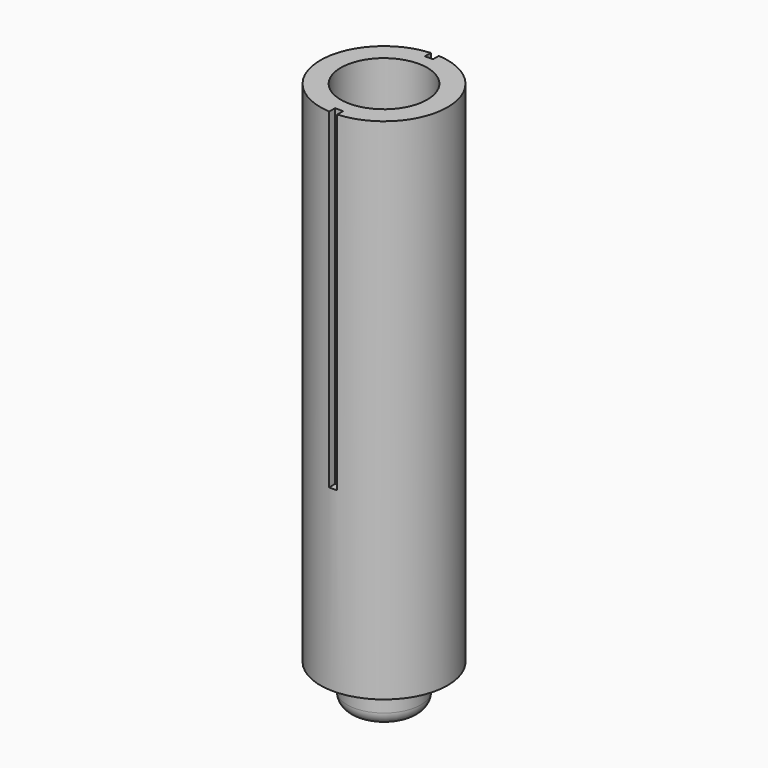
from build123d import *

# Parameters (mm, degrees)
F0_R     = 12.4999877
F0_R_2   = 8.4999957
F1_DEPTH = 100.000054
F0_R_3   = 7.2299957
F2_DEPTH = 5.08
F3_DEPTH = 29.99994
F5_DEPTH = 7.62
F6_R     = 2.54
F8_DEPTH = 65.000124


# Not quite as in the source:
# - a feature names something its author has since deleted; it is built from what else it names


with BuildPart() as f1:
    # F0 (on Top) → F1 (new body)
    with BuildSketch(Plane.XY):
        Circle(F0_R)
        Circle(F0_R_2, mode=Mode.SUBTRACT)
    extrude(amount=F1_DEPTH)

    # F0 (on Top) → F2 (join)
    with BuildSketch(Plane.XY):
        Circle(F0_R_2)
        Circle(F0_R_3, mode=Mode.SUBTRACT)
    extrude(amount=F2_DEPTH)

    # F0 (on Top) → F3 (join)
    with BuildSketch(Plane.XY):
        Circle(F0_R_2)
        Circle(F0_R_3, mode=Mode.SUBTRACT)
    extrude(amount=F3_DEPTH)

    # F7 (on face) → F8 (cut)
    with BuildSketch(Plane.XY.offset(100.000054)):
        Polygon((-0.7882758509, 11.0358614475), (0, 11.0358614475), (0.7882758509, 11.0358614475), (0.7882758509, 16.8001297861), (0, 16.8001297861), (-0.7882758509, 16.8001297861), align=None)
        Polygon((0, -11.0358614475), (-0.7882758509, -11.0358614475), (-0.7882758509, -16.8001297861), (0, -16.8001297861), (0.7882758509, -16.8001297861), (0.7882758509, -11.0358614475), align=None)
    extrude(amount=-F8_DEPTH, mode=Mode.SUBTRACT)


with BuildPart() as f5:
    # F0 (on Top) → F5 (new body)
    with BuildSketch(Plane.XY):
        Circle(F0_R_3)
    extrude(amount=-F5_DEPTH)

    # F6
    f6_edges = [f5.edges().sort_by_distance(p)[0] for p in [
        (-7.229996, 0, -7.62),
    ]]
    fillet(f6_edges, radius=F6_R)


solid = Compound([f1.part, f5.part])
